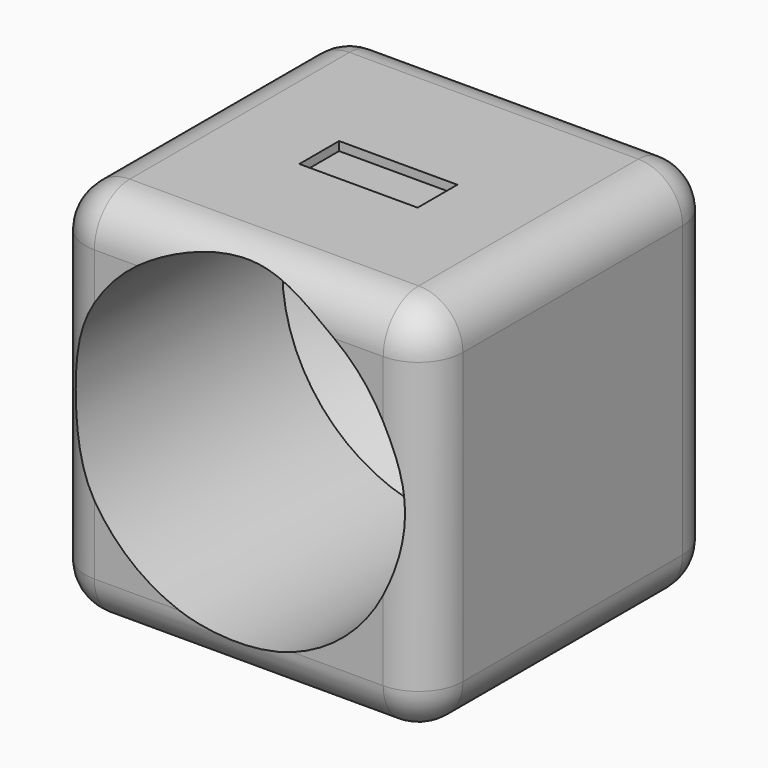
from build123d import *

# Parameters (mm, degrees)
F0_W         = 85.2558612823
F0_H         = 85.4500681162
F1_DEPTH     = 82
F3_D         = 75
F3_DEPTH     = 60
F3_TIP       = 22.5322732135
F4_R         = 10
F5_R         = 10
F6_R         = 10
F7_R         = 10
F8_T1_DEPTH  = 62
F8_T3_DEPTH  = 65.2558612823
F8_T5_DEPTH  = 65.4500681162
F8_S9_W      = 10
F8_S9_H      = 10
F8_T10_DEPTH = 10
F8_S15_W     = 10
F8_S15_H     = 10
F8_T16_DEPTH = 10
F8_T20_ANGLE = 90
F8_T22_ANGLE = 90
F8_T24_ANGLE = 90
F9_W         = 26.7179913353
F9_H         = 11.2215578556
F10_DEPTH    = 2


# Not quite as in the source:
# - a fillet or chamfer that OpenCascade refuses, or shapes differently, is made with other operations: its cross-section is extruded or revolved along the edge and cut away or added


with BuildPart() as f1:
    # F0 (on Front) → F1 (new body)
    with BuildSketch(Plane.XZ):
        with Locations((9.4189271331, 27.0915552974)):
            Rectangle(F0_W, F0_H)
    extrude(amount=F1_DEPTH)

    # F3
    with Locations(Plane.XZ.offset(82)):
        with Locations((8.7392125279, 29.616214335)):
            Hole(F3_D / 2, depth=F3_DEPTH)
            with Locations((0, 0, -(F3_DEPTH + F3_TIP / 2))):  # 118° drill point
                Cone(0, F3_D / 2, F3_TIP, mode=Mode.SUBTRACT)

    # F4
    f4_edges = [f1.edges().sort_by_distance(p)[0] for p in [
        (52.046858, -41, 69.816589),
    ]]
    fillet(f4_edges, radius=F4_R)

    # F5
    f5_edges = [f1.edges().sort_by_distance(p)[0] for p in [
        (-33.209004, -41, 69.816589),
    ]]
    fillet(f5_edges, radius=F5_R)

    # F6
    f6_edges = [f1.edges().sort_by_distance(p)[0] for p in [
        (52.046858, -41, -15.633479),
    ]]
    fillet(f6_edges, radius=F6_R)

    # F7
    f7_edges = [f1.edges().sort_by_distance(p)[0] for p in [
        (4.418927, 0, -15.633479),
    ]]
    fillet(f7_edges, radius=F7_R)

    # F8: fillet of radius 10 on 2 edges, made by hand

    # F8_s2 → F8_t1 (cut)
    with BuildSketch(Plane.XZ.offset(10)):
        with BuildLine():
            ThreePointArc((-23.2090035081, -15.6334787607), (-30.28007132, -12.7045465726), (-33.2090035081, -5.6334787607))
            Line((-33.2090035081, -5.6334787607), (-33.2090035081, -15.6334787607))
            Line((-33.2090035081, -15.6334787607), (-23.2090035081, -15.6334787607))
        make_face()
    extrude(amount=F8_T1_DEPTH, mode=Mode.SUBTRACT)

    # F8_s4 → F8_t3 (cut)
    with BuildSketch(Plane.YZ.offset(-23.2090035081)):
        with BuildLine():
            ThreePointArc((-72, 69.8165893555), (-79.0710678119, 66.8876571673), (-82, 59.8165893555))
            Line((-82, 59.8165893555), (-82, 69.8165893555))
            Line((-82, 69.8165893555), (-72, 69.8165893555))
        make_face()
        with BuildLine():
            ThreePointArc((-72, -15.6334787607), (-79.0710678119, -12.7045465726), (-82, -5.6334787607))
            Line((-82, -5.6334787607), (-82, -15.6334787607))
            Line((-82, -15.6334787607), (-72, -15.6334787607))
        make_face()
    extrude(amount=F8_T3_DEPTH, mode=Mode.SUBTRACT)

    # F8_s6 → F8_t5 (cut)
    with BuildSketch(Plane.XY.offset(-5.6334787607)):
        with BuildLine():
            ThreePointArc((-33.2090035081, -72), (-30.28007132, -79.0710678119), (-23.2090035081, -82))
            Line((-23.2090035081, -82), (-33.2090035081, -82))
            Line((-33.2090035081, -82), (-33.2090035081, -72))
        make_face()
        with BuildLine():
            ThreePointArc((52.0468577743, -72), (49.1179255861, -79.0710678119), (42.0468577743, -82))
            Line((42.0468577743, -82), (52.0468577743, -82))
            Line((52.0468577743, -82), (52.0468577743, -72))
        make_face()
    extrude(amount=F8_T5_DEPTH, mode=Mode.SUBTRACT)


with BuildPart() as f8_tool8:
    # F8_s9 → F8_t10 (new body)
    with BuildSketch(Plane.XY.offset(-5.6334787607)):
        with Locations((-28.2090035081, -5)):
            Rectangle(F8_S9_W, F8_S9_H)
    extrude(amount=-F8_T10_DEPTH)

    # F8_s11 → F8_t12 (revolve, cut)
    with BuildSketch(Plane(origin=(-23.2090035081, -10, -5.6334787607), x_dir=(0.7071067812, -0.7071067812, 0), z_dir=(0.7071067812, 0.7071067812, 0))):
        with BuildLine():
            ThreePointArc((0, -10), (10, 0), (0, 10))
            Line((0, 10), (0, -10))
        make_face()
    revolve(axis=Axis((-23.2090035081, -10, -5.6334787607), (0, 0, -1)), mode=Mode.SUBTRACT)


with BuildPart() as f1_1:
    add(f1.part)

    # F8_t7: cut F8_tool8
    add(f8_tool8.part, mode=Mode.SUBTRACT)


with BuildPart() as f8_tool14:
    # F8_s15 → F8_t16 (new body)
    with BuildSketch(Plane.YZ.offset(-23.2090035081)):
        with Locations((-77, -10.6334787607)):
            Rectangle(F8_S15_W, F8_S15_H)
    extrude(amount=-F8_T16_DEPTH)

    # F8_s17 → F8_t18 (revolve, cut)
    with BuildSketch(Plane(origin=(-23.2090035081, -72, -5.6334787607), x_dir=(0, 0.7071067812, 0.7071067812), z_dir=(0, -0.7071067812, 0.7071067812))):
        with BuildLine():
            ThreePointArc((0, -10), (10, 0), (0, 10))
            Line((0, 10), (0, -10))
        make_face()
    revolve(axis=Axis((-23.2090035081, -72, -5.6334787607), (-1, 0, 0)), mode=Mode.SUBTRACT)


with BuildPart() as f1_2:
    add(f1_1.part)

    # F8_t13: cut F8_tool14
    add(f8_tool14.part, mode=Mode.SUBTRACT)

    # F8_s19 → F8_t20 (revolve, cut)
    with BuildSketch(Plane.YZ.offset(42.0468577743)):
        with BuildLine():
            ThreePointArc((-82, 59.8165893555), (-79.0710678119, 66.8876571673), (-72, 69.8165893555))
            Line((-72, 69.8165893555), (-82, 69.8165893555))
            Line((-82, 69.8165893555), (-82, 59.8165893555))
        make_face()
    revolve(axis=Axis((42.0468577743, -82, 59.8165893555), (0, 1, 0)), revolution_arc=F8_T20_ANGLE, mode=Mode.SUBTRACT)

    # F8_s21 → F8_t22 (revolve, cut)
    with BuildSketch(Plane.YZ.offset(-23.2090035081)):
        with BuildLine():
            ThreePointArc((-82, 59.8165893555), (-79.0710678119, 66.8876571673), (-72, 69.8165893555))
            Line((-72, 69.8165893555), (-82, 69.8165893555))
            Line((-82, 69.8165893555), (-82, 59.8165893555))
        make_face()
    revolve(axis=Axis((-23.2090035081, -82, 59.8165893555), (0, -1, 0)), revolution_arc=F8_T22_ANGLE, mode=Mode.SUBTRACT)

    # F8_s23 → F8_t24 (revolve, cut)
    with BuildSketch(Plane.XY.offset(-5.6334787607)):
        with BuildLine():
            ThreePointArc((52.0468577743, -72), (49.1179255861, -79.0710678119), (42.0468577743, -82))
            Line((42.0468577743, -82), (52.0468577743, -82))
            Line((52.0468577743, -82), (52.0468577743, -72))
        make_face()
    revolve(axis=Axis((42.0468577743, -82, -5.6334787607), (0, 1, 0)), revolution_arc=F8_T24_ANGLE, mode=Mode.SUBTRACT)

    # F9 (on face) → F10 (cut)
    with BuildSketch(Plane.XY.offset(69.8165893555)):
        with Locations((9.8856553668, -43.1762188673)):
            Rectangle(F9_W, F9_H)
    extrude(amount=-F10_DEPTH, mode=Mode.SUBTRACT)


solid = f1_2.part
